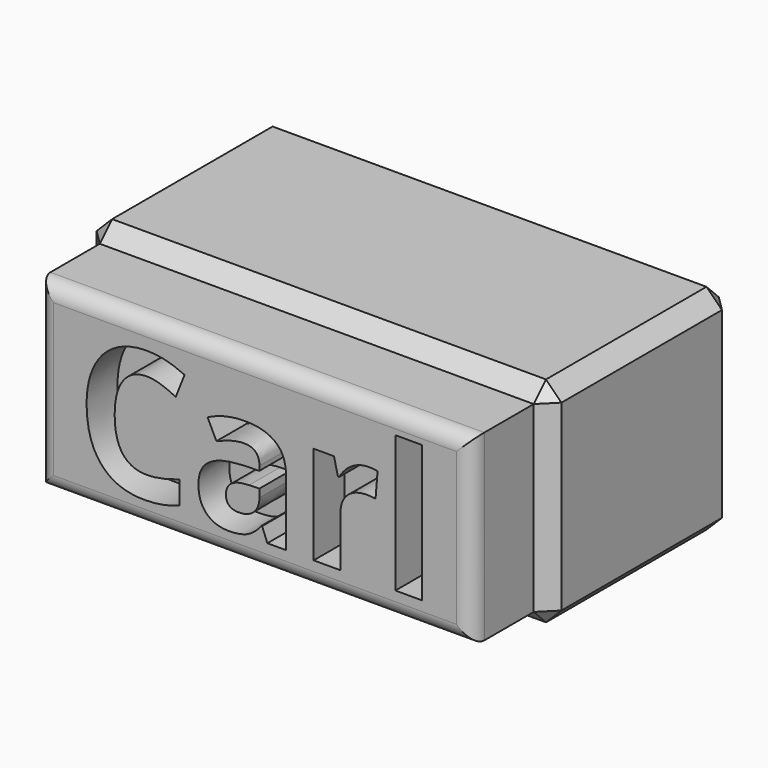
from build123d import *

# Parameters (mm, degrees)
F0_W         = 153.0096083879
F0_H         = 70.4087987542
F1_DEPTH     = 76.2
F2_SIZE      = 5.08
F3_DEPTH     = 25.4
F4_R         = 5.08
F5_TEXT_SIZE = 59.2666652261
F6_DEPTH     = 12.7


# Not quite as in the source:
# - Text() gives the source's letters only with a copy of the font that has no kerning and outlines rounded to 1/6400 em; it was checked with that copy


with BuildPart() as f1:
    # F0 (on Front) → F1 (new body)
    with BuildSketch(Plane.XZ):
        Rectangle(F0_W, F0_H)
    extrude(amount=F1_DEPTH)

    # F2
    f2_edges = [f1.edges().sort_by_distance(p)[0] for p in [
        (-76.504804, -38.1, 35.204399),
        (-76.504804, -38.1, -35.204399),
        (-76.504804, 0, 0),
        (-76.504804, -76.2, 0),
        (0, -76.2, 35.204399),
        (0, -76.2, -35.204399),
        (76.504804, -76.2, 0),
        (76.504804, -38.1, -35.204399),
        (76.504804, -38.1, 35.204399),
        (76.504804, 0, 0),
        (0, 0, 35.204399),
        (0, 0, -35.204399),
    ]]
    chamfer(f2_edges, length=F2_SIZE)

    # F3 (add): a face of the model
    f3_faces = [f1.faces().sort_by_distance(p)[0] for p in [
        (0, -76.2, 0),
    ]]
    extrude(f3_faces, amount=F3_DEPTH)

    # F4
    f4_edges = [f1.edges().sort_by_distance(p)[0] for p in [
        (0, -101.6, 30.124399),
        (0, -101.6, -30.124399),
        (-71.424804, -101.6, 0),
        (71.424804, -101.6, 0),
    ]]
    fillet(f4_edges, radius=F4_R)

    # F5 (on face) → F6 (cut)
    with BuildSketch(Plane.XZ.offset(101.6)):
        with Locations((-58.8843151927, -21.7931969091)):
            Text('Carl', F5_TEXT_SIZE, font='Open Sans', font_style=FontStyle.BOLD, text_align=(TextAlign.LEFT, TextAlign.BOTTOM))
    extrude(amount=-F6_DEPTH, mode=Mode.SUBTRACT)


solid = f1.part
